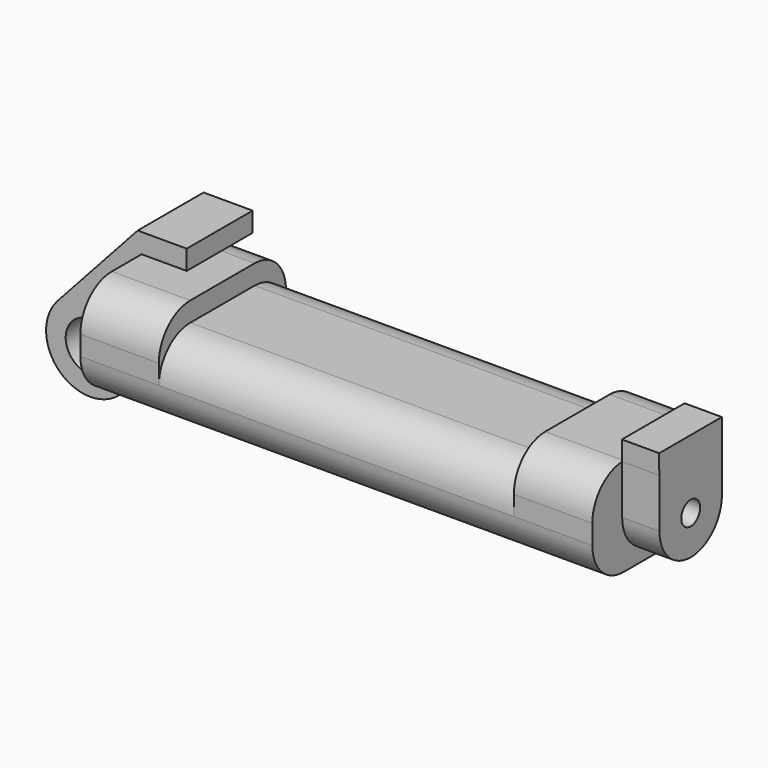
from build123d import *

# Parameters (mm, degrees)
F0_W     = 5.842
F0_H     = 12.7
F1_DEPTH = 20.574
F2_R     = 5.08
F3_R     = 5.07999
F0_R     = 3.175
F4_DEPTH = 10.668
F5_R     = 1.5253482573
F6_DEPTH = 4.826


# Not quite as in the source:
# - a fillet or chamfer is up to 0.001 mm smaller than in the source, because OpenCascade refuses the exact size


with BuildPart() as f1:
    # F0 (on Front) → F1 (new body)
    with BuildSketch(Plane.XZ):
        Polygon((5.842, 12.7), (5.842, 0), (66.294, 0), (66.294, 12.7), (56.134, 12.7), (56.134, 10.16), (10.16, 10.16), (10.16, 12.7), align=None)
        with Locations((2.921, 6.35)):
            Rectangle(F0_W, F0_H)
    extrude(amount=F1_DEPTH)

    # F2
    f2_edges = [f1.edges().sort_by_distance(p)[0] for p in [
        (33.147, 0, 10.16),
        (33.147, -20.574, 10.16),
    ]]
    fillet(f2_edges, radius=F2_R)

    # F3 (radius 5.08 in the source; OpenCascade refuses exactly that, so slightly less here)
    f3_edges = [f1.edges().sort_by_distance(p)[0] for p in [
        (33.147, 0, 0),
        (61.214, 0, 12.7),
        (61.214, -20.574, 12.7),
        (5.08, 0, 12.7),
        (5.08, -20.574, 12.7),
        (33.147, -20.574, 0),
    ]]
    fillet(f3_edges, radius=F3_R)

    # F0 (on Front) → F4 (join)
    with BuildSketch(Plane.XZ):
        with BuildLine():
            ThreePointArc((-8.1826630726, -5.5069827884), (-3.1957909266, -4.5493385486), (-0.9398, 0))
            ThreePointArc((-0.9398, 0), (-4.5919612295, 5.3297205562), (-10.8806298187, 3.8475430269))
            ThreePointArc((-10.8806298187, 3.8475430269), (-12.1459778134, -1.5837270034), (-8.1826630726, -5.5069827884))
        make_face()
        with Locations((-6.6548, 0)):
            Circle(F0_R, mode=Mode.SUBTRACT)
        with BuildLine():
            Line((-0.9398, 0), (0, 0))
            Line((0, 0), (0, 12.7))
            Line((0, 12.7), (5.842, 12.7))
            Line((5.842, 12.7), (5.842, 15.24))
            Line((5.842, 15.24), (-0.508, 15.24))
            Line((-0.508, 15.24), (-10.8806298187, 3.8475430269))
            ThreePointArc((-10.8806298187, 3.8475430269), (-4.5919612295, 5.3297205562), (-0.9398, 0))
        make_face()
    extrude(amount=F4_DEPTH)

    # F5 (on face) → F6 (join)
    with BuildSketch(Plane.YZ.offset(66.294)):
        with BuildLine():
            Line((-15.49401, 12.7), (-5.6335453628, 12.7))
            Line((-5.6335453628, 12.7), (-5.6335453628, 15.2267941305))
            Line((-5.6335453628, 15.2267941305), (-14.7798256949, 15.2267941305))
            Line((-14.7798256949, 15.2267941305), (-15.7828871161, 15.2267941305))
            Line((-15.7828871161, 15.2267941305), (-15.7713881355, 12.6924216326))
            ThreePointArc((-15.7713881355, 12.6924216326), (-15.632750821, 12.6981050547), (-15.49401, 12.7))
        make_face()
        with BuildLine():
            ThreePointArc((-15.7424642816, 6.3176113686), (-10.7967240539, 11.3957731119), (-5.6335453628, 6.5388544493))
            Line((-5.6335453628, 6.5388544493), (-5.6335453628, 12.7))
            Line((-5.6335453628, 12.7), (-15.49401, 12.7))
            ThreePointArc((-15.49401, 12.7), (-15.632750821, 12.6981050547), (-15.7713881355, 12.6924216326))
            Line((-15.7713881355, 12.6924216326), (-15.7424642816, 6.3176113686))
        make_face()
        with BuildLine():
            ThreePointArc((-15.7424642816, 6.3176113686), (-10.6746149155, 1.2841357749), (-5.6296554142, 6.3405532201))
            ThreePointArc((-5.6296554142, 6.3405532201), (-5.6306279949, 6.4397229095), (-5.6335453628, 6.5388544493))
            ThreePointArc((-5.6335453628, 6.5388544493), (-10.7967240539, 11.3957731119), (-15.7424642816, 6.3176113686))
        make_face()
        with Locations((-10.6860858708, 6.3405532201)):
            Circle(F5_R, mode=Mode.SUBTRACT)
    extrude(amount=F6_DEPTH)


solid = f1.part
